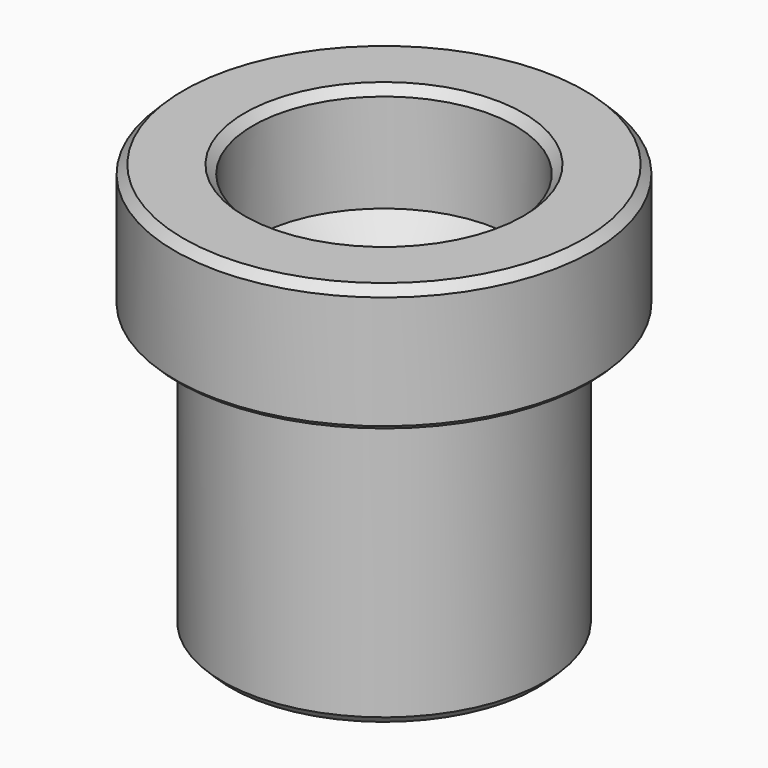
from build123d import *

# Parameters (mm, degrees)
F2_SIZE     = 0.254
F3_S5_R     = 3.96875
F3_T6_DEPTH = 9
F4_SIZE     = 0.127


# Not quite as in the source:
# - a fillet or chamfer that OpenCascade refuses, or shapes differently, is made with other operations: its cross-section is extruded or revolved along the edge and cut away or added


with BuildPart() as f1:
    # F0 (on Front) → F1 (revolve)
    with BuildSketch(Plane.XZ):
        Polygon((6.3246, -3.81), (6.3246, 0), (3.96875, 0), (3.96875, -2.159), (2.50825, -2.159), (2.50825, -12.446), (4.8895, -12.446), (4.8895, -3.81), align=None)
    revolve(axis=Axis((0, 0, -10.7170343399), (0, 0, -1)))

    # F2
    f2_edges = [f1.edges().sort_by_distance(p)[0] for p in [
        (-6.3246, 0, 0),
        (-4.8895, 0, -12.446),
        (-2.50825, 0, -12.446),
        (-3.96875, 0, 0),
    ]]
    chamfer(f2_edges, length=F2_SIZE)

    # F3: chamfer of 2.54 on 1 edges, made by hand


with BuildPart() as f3_tool2:
    # F3_s3 → F3_t4 (revolve)
    with BuildSketch(Plane.XZ):
        Polygon((2.50825, -4.699), (5.04825, -2.159), (2.50825, -2.159), align=None)
    revolve(axis=Axis((0, 0, -2.159), (0, 0, -1)))

    # F3_s5 → F3_t6 (intersect, symmetric)
    with BuildSketch(Plane.XY.offset(-3.4)):
        Circle(F3_S5_R)
    extrude(amount=F3_T6_DEPTH, both=True, mode=Mode.INTERSECT)


with BuildPart() as f1_1:
    add(f1.part)

    # F3_t1: cut F3_tool2
    add(f3_tool2.part, mode=Mode.SUBTRACT)

    # F4
    f4_edges = [f1_1.edges().sort_by_distance(p)[0] for p in [
        (-6.3246, 0, -3.81),
    ]]
    chamfer(f4_edges, length=F4_SIZE)


solid = f1_1.part
